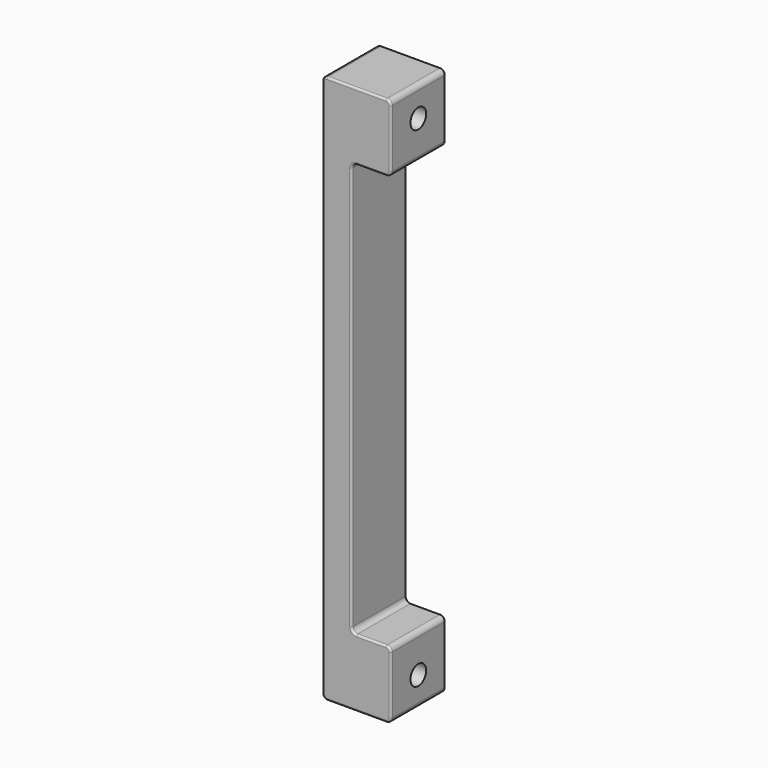
from build123d import *

# Parameters (mm, degrees)
F0_R     = 1
F1_DEPTH = 7
F0_W     = 7
F0_H     = 42.2
F2_DEPTH = 3
F3_R     = 0.5
F4_R     = 0.2


with BuildPart() as f1:
    # F0 (on Right) → F1 (new body)
    with BuildSketch(Plane.YZ):
        Polygon((3.5, -22.5), (3.5, -21.1), (-3.5, -21.1), (-3.5, -22.5), (-3.5, -28), (3.5, -28), align=None)
        with Locations((0, -25)):
            Circle(F0_R, mode=Mode.SUBTRACT)
    extrude(amount=F1_DEPTH)



with BuildPart() as f1b:
    # F0 (on Right) → F1, piece 2 (new body)
    with BuildSketch(Plane.YZ):
        Polygon((3.5, 22.5), (3.5, 28), (-3.5, 28), (-3.5, 22.5), (-3.5, 21.1), (3.5, 21.1), align=None)
        with Locations((0, 25)):
            Circle(F0_R, mode=Mode.SUBTRACT)
    extrude(amount=F1_DEPTH)


with BuildPart() as f1_1:
    add(f1.part)

    add(f1b.part)  # F2 merges F1b
    # F0 (on Right) → F2 (join)
    with BuildSketch(Plane.YZ):
        Rectangle(F0_W, F0_H)
    extrude(amount=F2_DEPTH)

    # F3
    f3_edges = [f1_1.edges().sort_by_distance(p)[0] for p in [
        (7, 0, -21.1),
        (7, 0, -28),
        (7, 0, 21.1),
        (7, 0, 28),
        (0, 0, 28),
        (0, 0, -28),
        (3, 0, 21.1),
        (3, 0, -21.1),
    ]]
    fillet(f3_edges, radius=F3_R)

    # F4
    f4_edges = [f1_1.edges().sort_by_distance(p)[0] for p in [
        (3, 3.5, 0),
        (3, -3.5, 0),
        (3.5, 3.5, 28),
        (0.146447, 3.5, 27.853553),
        (6.853553, 3.5, 27.853553),
        (0, 3.5, 0),
        (7, 3.5, 24.55),
        (0.146447, 3.5, -27.853553),
        (6.853553, 3.5, 21.246447),
        (3.5, 3.5, -28),
        (5, 3.5, 21.1),
        (6.853553, 3.5, -27.853553),
        (3.146447, 3.5, 20.953553),
        (7, 3.5, -24.55),
        (6.853553, 3.5, -21.246447),
        (3.146447, 3.5, -20.953553),
        (5, 3.5, -21.1),
        (3.5, -3.5, 28),
        (0.146447, -3.5, 27.853553),
        (6.853553, -3.5, 27.853553),
        (0, -3.5, 0),
        (7, -3.5, 24.55),
        (0.146447, -3.5, -27.853553),
        (6.853553, -3.5, 21.246447),
        (3.5, -3.5, -28),
        (5, -3.5, 21.1),
        (6.853553, -3.5, -27.853553),
        (3.146447, -3.5, 20.953553),
        (7, -3.5, -24.55),
        (6.853553, -3.5, -21.246447),
        (3.146447, -3.5, -20.953553),
        (5, -3.5, -21.1),
    ]]
    fillet(f4_edges, radius=F4_R)


solid = f1_1.part
